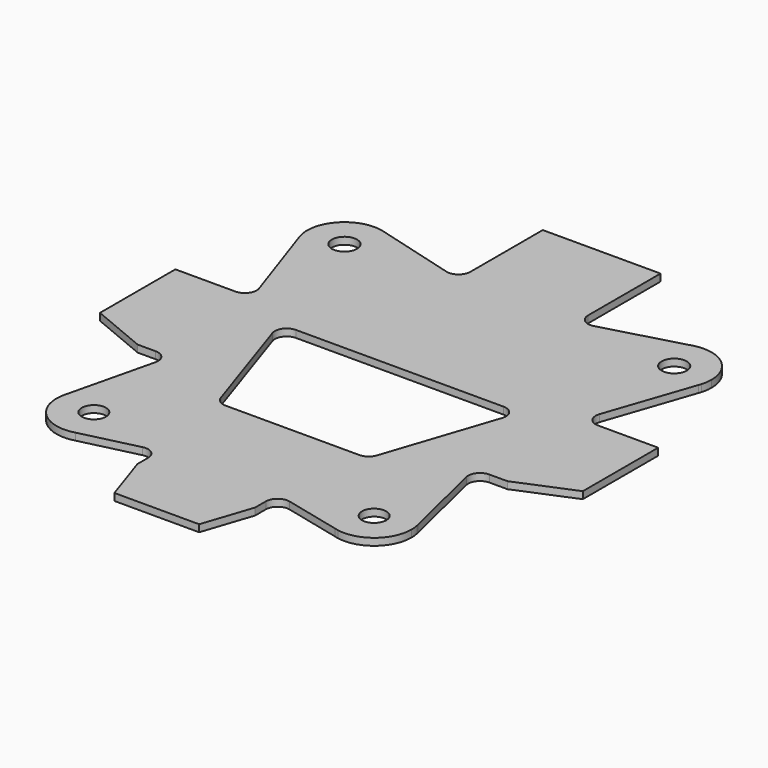
from build123d import *

# Parameters (mm, degrees)
F0_R     = 5.15
F0_R_2   = 5.35
F1_DEPTH = 3
F2_DEPTH = 3


# Not quite as in the source:
# - a feature names something its author has since deleted; it is built from what else it names


with BuildPart() as f1:
    # F0 (on Top) → F1 (new body)
    with BuildSketch(Plane.XY):
        with BuildLine():
            Line((-25, -20), (0, -20))
            Line((0, -20), (25, -20))
            Line((25, -20), (25, -14.3424324172))
            ThreePointArc((25, -14.3424324172), (26.9045190123, -10.4158566246), (31.167198982, -9.4805761322))
            Line((31.167198982, -9.4805761322), (55.0829571834, -15.2220968581))
            ThreePointArc((55.0829571834, -15.2220968581), (48.4016498049, 11.3158792388), (74.8049560197, 4.1207792025))
            Line((74.8049560197, 4.1207792025), (65.9824120319, 40.8316405516))
            ThreePointArc((65.9824120319, 40.8316405516), (66.917044372, 45.0950123391), (70.8439895742, 47))
            Line((70.8439895742, 47), (78.5, 47))
            Line((78.5, 47), (102.5, 57))
            Line((102.5, 57), (102.5, 97))
            Line((102.5, 97), (78.5, 97))
            Line((78.5, 97), (76.9853890649, 97))
            ThreePointArc((76.9853890649, 97), (72.9195967319, 99.0897882028), (72.2524623398, 103.6122669181))
            Line((72.2524623398, 103.6122669181), (84.8119254692, 140.4814838147))
            ThreePointArc((84.8119254692, 140.4814838147), (58.3240216641, 135.4043723862), (65.6425820254, 161.362507579))
            Line((65.6425820254, 161.362507579), (31.3326776693, 151.8744700251))
            ThreePointArc((31.3326776693, 151.8744700251), (26.9720789596, 152.7146893354), (25, 156.6935954883))
            Line((25, 156.6935954883), (25, 195.1232356609))
            Line((25, 195.1232356609), (0, 195.1232356609))
            Line((0, 195.1232356609), (-25, 195.1232356609))
            Line((-25, 195.1232356609), (-25, 156.6935954883))
            ThreePointArc((-25, 156.6935954883), (-26.9720789596, 152.7146893354), (-31.3326776693, 151.8744700251))
            Line((-31.3326776693, 151.8744700251), (-65.6425820254, 161.362507579))
            ThreePointArc((-65.6425820254, 161.362507579), (-57.3452069377, 155.666752442), (-54.15, 146.1232356609))
            ThreePointArc((-54.15, 146.1232356609), (-67.1317704666, 130.5349144124), (-84.8119254692, 140.4814838147))
            Line((-84.8119254692, 140.4814838147), (-72.2524623398, 103.6122669181))
            ThreePointArc((-72.2524623398, 103.6122669181), (-72.9195967319, 99.0897882028), (-76.9853890649, 97))
            Line((-76.9853890649, 97), (-78.5, 97))
            Line((-78.5, 97), (-102.5, 97))
            Line((-102.5, 97), (-102.5, 57))
            Line((-102.5, 57), (-78.5, 47))
            Line((-78.5, 47), (-70.8439895742, 47))
            ThreePointArc((-70.8439895742, 47), (-66.917044372, 45.0950123391), (-65.9824120319, 40.8316405516))
            Line((-65.9824120319, 40.8316405516), (-74.8049560197, 4.1207792025))
            ThreePointArc((-74.8049560197, 4.1207792025), (-57.4216656804, 15.7131482032), (-43.65, 0))
            ThreePointArc((-43.65, 0), (-46.826550812, -9.5187281545), (-55.0829571834, -15.2220968581))
            Line((-55.0829571834, -15.2220968581), (-31.167198982, -9.4805761322))
            ThreePointArc((-31.167198982, -9.4805761322), (-26.9045190123, -10.4158566246), (-25, -14.3424324172))
            Line((-25, -14.3424324172), (-25, -20))
        make_face()
        with BuildLine():
            Line((28.3962038997, 31), (0, 31))
            Line((0, 31), (-28.3962038997, 31))
            ThreePointArc((-28.3962038997, 31), (-31.319755323, 31.9437890741), (-33.13962039, 34.4188611699))
            Line((-33.13962039, 34.4188611699), (-48.8062870566, 81.4188611699))
            ThreePointArc((-48.8062870566, 81.4188611699), (-48.1190814923, 85.9235514233), (-44.0628705664, 88))
            Line((-44.0628705664, 88), (0, 88))
            Line((0, 88), (44.0628705664, 88))
            ThreePointArc((44.0628705664, 88), (48.1190814923, 85.9235514233), (48.8062870566, 81.4188611699))
            Line((48.8062870566, 81.4188611699), (33.13962039, 34.4188611699))
            ThreePointArc((33.13962039, 34.4188611699), (31.319755323, 31.9437890741), (28.3962038997, 31))
        make_face(mode=Mode.SUBTRACT)
        Polygon((25, -20), (0, -20), (-25, -20), (-18, -41), (0, -41), (18, -41), align=None)
        with BuildLine():
            ThreePointArc((74.8049560197, 4.1207792025), (48.4016498049, 11.3158792388), (55.0829571834, -15.2220968581))
            Line((55.0829571834, -15.2220968581), (56.5251048848, -15.5683171555))
            Line((56.5251048848, -15.5683171555), (75.0060818693, 3.2838887103))
            Line((75.0060818693, 3.2838887103), (74.8049560197, 4.1207792025))
        make_face()
        with Locations((59.5, 0)):
            Circle(F0_R, mode=Mode.SUBTRACT)
        with BuildLine():
            Line((56.5251048848, -15.5683171555), (55.0829571834, -15.2220968581))
            ThreePointArc((55.0829571834, -15.2220968581), (55.799979227, -15.4120844236), (56.5251048848, -15.5683171555))
        make_face()
        with BuildLine():
            Line((-56.5251048848, -15.5683171555), (-55.0829571834, -15.2220968581))
            ThreePointArc((-55.0829571834, -15.2220968581), (-46.826550812, -9.5187281545), (-43.65, 0))
            ThreePointArc((-43.65, 0), (-57.4216656804, 15.7131482032), (-74.8049560197, 4.1207792025))
            Line((-74.8049560197, 4.1207792025), (-75.0060818693, 3.2838887103))
            Line((-75.0060818693, 3.2838887103), (-56.5251048848, -15.5683171555))
        make_face()
        with Locations((-59.5, 0)):
            Circle(F0_R, mode=Mode.SUBTRACT)
        with BuildLine():
            ThreePointArc((-56.5251048848, -15.5683171555), (-55.799979227, -15.4120844236), (-55.0829571834, -15.2220968581))
            Line((-55.0829571834, -15.2220968581), (-56.5251048848, -15.5683171555))
        make_face()
        with BuildLine():
            Line((75.0060818693, 3.2838887103), (56.5251048848, -15.5683171555))
            ThreePointArc((56.5251048848, -15.5683171555), (69.6012477552, -12.2142250588), (75.35, 0))
            ThreePointArc((75.35, 0), (75.2637859924, 1.6509243428), (75.0060818693, 3.2838887103))
        make_face()
        with BuildLine():
            ThreePointArc((75.0060818693, 3.2838887103), (74.9112008089, 3.7036994515), (74.8049560197, 4.1207792025))
            Line((74.8049560197, 4.1207792025), (75.0060818693, 3.2838887103))
        make_face()
        with BuildLine():
            ThreePointArc((-75.0060818693, 3.2838887103), (-70.8185280345, -11.0956488378), (-56.5251048848, -15.5683171555))
            Line((-56.5251048848, -15.5683171555), (-75.0060818693, 3.2838887103))
        make_face()
        with BuildLine():
            ThreePointArc((-74.8049560197, 4.1207792025), (-74.9112008089, 3.7036994515), (-75.0060818693, 3.2838887103))
            Line((-75.0060818693, 3.2838887103), (-74.8049560197, 4.1207792025))
        make_face()
        with BuildLine():
            ThreePointArc((65.6425820254, 161.362507579), (58.3240216641, 135.4043723862), (84.8119254692, 140.4814838147))
            Line((84.8119254692, 140.4814838147), (85.1758103286, 141.5496942681))
            Line((85.1758103286, 141.5496942681), (65.9085617168, 161.4360614215))
            Line((65.9085617168, 161.4360614215), (65.6425820254, 161.362507579))
        make_face()
        with Locations((70, 146.1232356609)):
            Circle(F0_R_2, mode=Mode.SUBTRACT)
        with BuildLine():
            Line((85.1758103286, 141.5496942681), (84.8119254692, 140.4814838147))
            ThreePointArc((84.8119254692, 140.4814838147), (85.0033777185, 141.0123495306), (85.1758103286, 141.5496942681))
        make_face()
        with BuildLine():
            Line((65.9085617168, 161.4360614215), (85.1758103286, 141.5496942681))
            ThreePointArc((85.1758103286, 141.5496942681), (85.6805467651, 143.8117527719), (85.85, 146.1232356609))
            ThreePointArc((85.85, 146.1232356609), (79.6533207553, 158.6944686312), (65.9085617168, 161.4360614215))
        make_face()
        with BuildLine():
            ThreePointArc((65.9085617168, 161.4360614215), (65.7754117883, 161.3998633791), (65.6425820254, 161.362507579))
            Line((65.6425820254, 161.362507579), (65.9085617168, 161.4360614215))
        make_face()
        with BuildLine():
            ThreePointArc((-85.1758103286, 141.5496942681), (-85.0033777185, 141.0123495306), (-84.8119254692, 140.4814838147))
            Line((-84.8119254692, 140.4814838147), (-85.1758103286, 141.5496942681))
        make_face()
        with BuildLine():
            Line((-85.1758103286, 141.5496942681), (-84.8119254692, 140.4814838147))
            ThreePointArc((-84.8119254692, 140.4814838147), (-67.1317704666, 130.5349144124), (-54.15, 146.1232356609))
            ThreePointArc((-54.15, 146.1232356609), (-57.3452069377, 155.666752442), (-65.6425820254, 161.362507579))
            Line((-65.6425820254, 161.362507579), (-65.9085617168, 161.4360614215))
            Line((-65.9085617168, 161.4360614215), (-85.1758103286, 141.5496942681))
        make_face()
        with Locations((-70, 146.1232356609)):
            Circle(F0_R_2, mode=Mode.SUBTRACT)
        with BuildLine():
            ThreePointArc((-65.9085617168, 161.4360614215), (-81.3834408484, 157.1522779788), (-85.1758103286, 141.5496942681))
            Line((-85.1758103286, 141.5496942681), (-65.9085617168, 161.4360614215))
        make_face()
        with BuildLine():
            ThreePointArc((-65.6425820254, 161.362507579), (-65.7754117883, 161.3998633791), (-65.9085617168, 161.4360614215))
            Line((-65.9085617168, 161.4360614215), (-65.6425820254, 161.362507579))
        make_face()
    extrude(amount=F1_DEPTH)

    # F0 (on Top) → F2 (join)
    with BuildSketch(Plane.XY):
        with BuildLine():
            Line((-25, -20), (0, -20))
            Line((0, -20), (25, -20))
            Line((25, -20), (25, -14.3424324172))
            ThreePointArc((25, -14.3424324172), (26.9045190123, -10.4158566246), (31.167198982, -9.4805761322))
            Line((31.167198982, -9.4805761322), (55.0829571834, -15.2220968581))
            ThreePointArc((55.0829571834, -15.2220968581), (48.4016498049, 11.3158792388), (74.8049560197, 4.1207792025))
            Line((74.8049560197, 4.1207792025), (65.9824120319, 40.8316405516))
            ThreePointArc((65.9824120319, 40.8316405516), (66.917044372, 45.0950123391), (70.8439895742, 47))
            Line((70.8439895742, 47), (78.5, 47))
            Line((78.5, 47), (102.5, 57))
            Line((102.5, 57), (102.5, 97))
            Line((102.5, 97), (78.5, 97))
            Line((78.5, 97), (76.9853890649, 97))
            ThreePointArc((76.9853890649, 97), (72.9195967319, 99.0897882028), (72.2524623398, 103.6122669181))
            Line((72.2524623398, 103.6122669181), (84.8119254692, 140.4814838147))
            ThreePointArc((84.8119254692, 140.4814838147), (58.3240216641, 135.4043723862), (65.6425820254, 161.362507579))
            Line((65.6425820254, 161.362507579), (31.3326776693, 151.8744700251))
            ThreePointArc((31.3326776693, 151.8744700251), (26.9720789596, 152.7146893354), (25, 156.6935954883))
            Line((25, 156.6935954883), (25, 195.1232356609))
            Line((25, 195.1232356609), (0, 195.1232356609))
            Line((0, 195.1232356609), (-25, 195.1232356609))
            Line((-25, 195.1232356609), (-25, 156.6935954883))
            ThreePointArc((-25, 156.6935954883), (-26.9720789596, 152.7146893354), (-31.3326776693, 151.8744700251))
            Line((-31.3326776693, 151.8744700251), (-65.6425820254, 161.362507579))
            ThreePointArc((-65.6425820254, 161.362507579), (-57.3452069377, 155.666752442), (-54.15, 146.1232356609))
            ThreePointArc((-54.15, 146.1232356609), (-67.1317704666, 130.5349144124), (-84.8119254692, 140.4814838147))
            Line((-84.8119254692, 140.4814838147), (-72.2524623398, 103.6122669181))
            ThreePointArc((-72.2524623398, 103.6122669181), (-72.9195967319, 99.0897882028), (-76.9853890649, 97))
            Line((-76.9853890649, 97), (-78.5, 97))
            Line((-78.5, 97), (-102.5, 97))
            Line((-102.5, 97), (-102.5, 57))
            Line((-102.5, 57), (-78.5, 47))
            Line((-78.5, 47), (-70.8439895742, 47))
            ThreePointArc((-70.8439895742, 47), (-66.917044372, 45.0950123391), (-65.9824120319, 40.8316405516))
            Line((-65.9824120319, 40.8316405516), (-74.8049560197, 4.1207792025))
            ThreePointArc((-74.8049560197, 4.1207792025), (-57.4216656804, 15.7131482032), (-43.65, 0))
            ThreePointArc((-43.65, 0), (-46.826550812, -9.5187281545), (-55.0829571834, -15.2220968581))
            Line((-55.0829571834, -15.2220968581), (-31.167198982, -9.4805761322))
            ThreePointArc((-31.167198982, -9.4805761322), (-26.9045190123, -10.4158566246), (-25, -14.3424324172))
            Line((-25, -14.3424324172), (-25, -20))
        make_face()
        with BuildLine():
            Line((28.3962038997, 31), (0, 31))
            Line((0, 31), (-28.3962038997, 31))
            ThreePointArc((-28.3962038997, 31), (-31.319755323, 31.9437890741), (-33.13962039, 34.4188611699))
            Line((-33.13962039, 34.4188611699), (-48.8062870566, 81.4188611699))
            ThreePointArc((-48.8062870566, 81.4188611699), (-48.1190814923, 85.9235514233), (-44.0628705664, 88))
            Line((-44.0628705664, 88), (0, 88))
            Line((0, 88), (44.0628705664, 88))
            ThreePointArc((44.0628705664, 88), (48.1190814923, 85.9235514233), (48.8062870566, 81.4188611699))
            Line((48.8062870566, 81.4188611699), (33.13962039, 34.4188611699))
            ThreePointArc((33.13962039, 34.4188611699), (31.319755323, 31.9437890741), (28.3962038997, 31))
        make_face(mode=Mode.SUBTRACT)
        Polygon((25, -20), (0, -20), (-25, -20), (-18, -41), (0, -41), (18, -41), align=None)
        with BuildLine():
            ThreePointArc((74.8049560197, 4.1207792025), (48.4016498049, 11.3158792388), (55.0829571834, -15.2220968581))
            Line((55.0829571834, -15.2220968581), (56.5251048848, -15.5683171555))
            Line((56.5251048848, -15.5683171555), (75.0060818693, 3.2838887103))
            Line((75.0060818693, 3.2838887103), (74.8049560197, 4.1207792025))
        make_face()
        with Locations((59.5, 0)):
            Circle(F0_R, mode=Mode.SUBTRACT)
        with BuildLine():
            Line((56.5251048848, -15.5683171555), (55.0829571834, -15.2220968581))
            ThreePointArc((55.0829571834, -15.2220968581), (55.799979227, -15.4120844236), (56.5251048848, -15.5683171555))
        make_face()
        with BuildLine():
            Line((-56.5251048848, -15.5683171555), (-55.0829571834, -15.2220968581))
            ThreePointArc((-55.0829571834, -15.2220968581), (-46.826550812, -9.5187281545), (-43.65, 0))
            ThreePointArc((-43.65, 0), (-57.4216656804, 15.7131482032), (-74.8049560197, 4.1207792025))
            Line((-74.8049560197, 4.1207792025), (-75.0060818693, 3.2838887103))
            Line((-75.0060818693, 3.2838887103), (-56.5251048848, -15.5683171555))
        make_face()
        with Locations((-59.5, 0)):
            Circle(F0_R, mode=Mode.SUBTRACT)
        with BuildLine():
            ThreePointArc((-56.5251048848, -15.5683171555), (-55.799979227, -15.4120844236), (-55.0829571834, -15.2220968581))
            Line((-55.0829571834, -15.2220968581), (-56.5251048848, -15.5683171555))
        make_face()
        with BuildLine():
            Line((75.0060818693, 3.2838887103), (56.5251048848, -15.5683171555))
            ThreePointArc((56.5251048848, -15.5683171555), (69.6012477552, -12.2142250588), (75.35, 0))
            ThreePointArc((75.35, 0), (75.2637859924, 1.6509243428), (75.0060818693, 3.2838887103))
        make_face()
        with BuildLine():
            ThreePointArc((75.0060818693, 3.2838887103), (74.9112008089, 3.7036994515), (74.8049560197, 4.1207792025))
            Line((74.8049560197, 4.1207792025), (75.0060818693, 3.2838887103))
        make_face()
        with BuildLine():
            ThreePointArc((-75.0060818693, 3.2838887103), (-70.8185280345, -11.0956488378), (-56.5251048848, -15.5683171555))
            Line((-56.5251048848, -15.5683171555), (-75.0060818693, 3.2838887103))
        make_face()
        with BuildLine():
            ThreePointArc((-74.8049560197, 4.1207792025), (-74.9112008089, 3.7036994515), (-75.0060818693, 3.2838887103))
            Line((-75.0060818693, 3.2838887103), (-74.8049560197, 4.1207792025))
        make_face()
        with BuildLine():
            ThreePointArc((65.6425820254, 161.362507579), (58.3240216641, 135.4043723862), (84.8119254692, 140.4814838147))
            Line((84.8119254692, 140.4814838147), (85.1758103286, 141.5496942681))
            Line((85.1758103286, 141.5496942681), (65.9085617168, 161.4360614215))
            Line((65.9085617168, 161.4360614215), (65.6425820254, 161.362507579))
        make_face()
        with Locations((70, 146.1232356609)):
            Circle(F0_R_2, mode=Mode.SUBTRACT)
        with BuildLine():
            Line((85.1758103286, 141.5496942681), (84.8119254692, 140.4814838147))
            ThreePointArc((84.8119254692, 140.4814838147), (85.0033777185, 141.0123495306), (85.1758103286, 141.5496942681))
        make_face()
        with BuildLine():
            Line((65.9085617168, 161.4360614215), (85.1758103286, 141.5496942681))
            ThreePointArc((85.1758103286, 141.5496942681), (85.6805467651, 143.8117527719), (85.85, 146.1232356609))
            ThreePointArc((85.85, 146.1232356609), (79.6533207553, 158.6944686312), (65.9085617168, 161.4360614215))
        make_face()
        with BuildLine():
            ThreePointArc((65.9085617168, 161.4360614215), (65.7754117883, 161.3998633791), (65.6425820254, 161.362507579))
            Line((65.6425820254, 161.362507579), (65.9085617168, 161.4360614215))
        make_face()
        with BuildLine():
            ThreePointArc((-85.1758103286, 141.5496942681), (-85.0033777185, 141.0123495306), (-84.8119254692, 140.4814838147))
            Line((-84.8119254692, 140.4814838147), (-85.1758103286, 141.5496942681))
        make_face()
        with BuildLine():
            Line((-85.1758103286, 141.5496942681), (-84.8119254692, 140.4814838147))
            ThreePointArc((-84.8119254692, 140.4814838147), (-67.1317704666, 130.5349144124), (-54.15, 146.1232356609))
            ThreePointArc((-54.15, 146.1232356609), (-57.3452069377, 155.666752442), (-65.6425820254, 161.362507579))
            Line((-65.6425820254, 161.362507579), (-65.9085617168, 161.4360614215))
            Line((-65.9085617168, 161.4360614215), (-85.1758103286, 141.5496942681))
        make_face()
        with Locations((-70, 146.1232356609)):
            Circle(F0_R_2, mode=Mode.SUBTRACT)
        with BuildLine():
            ThreePointArc((-65.9085617168, 161.4360614215), (-81.3834408484, 157.1522779788), (-85.1758103286, 141.5496942681))
            Line((-85.1758103286, 141.5496942681), (-65.9085617168, 161.4360614215))
        make_face()
        with BuildLine():
            ThreePointArc((-65.6425820254, 161.362507579), (-65.7754117883, 161.3998633791), (-65.9085617168, 161.4360614215))
            Line((-65.9085617168, 161.4360614215), (-65.6425820254, 161.362507579))
        make_face()
    extrude(amount=F2_DEPTH)


solid = f1.part
